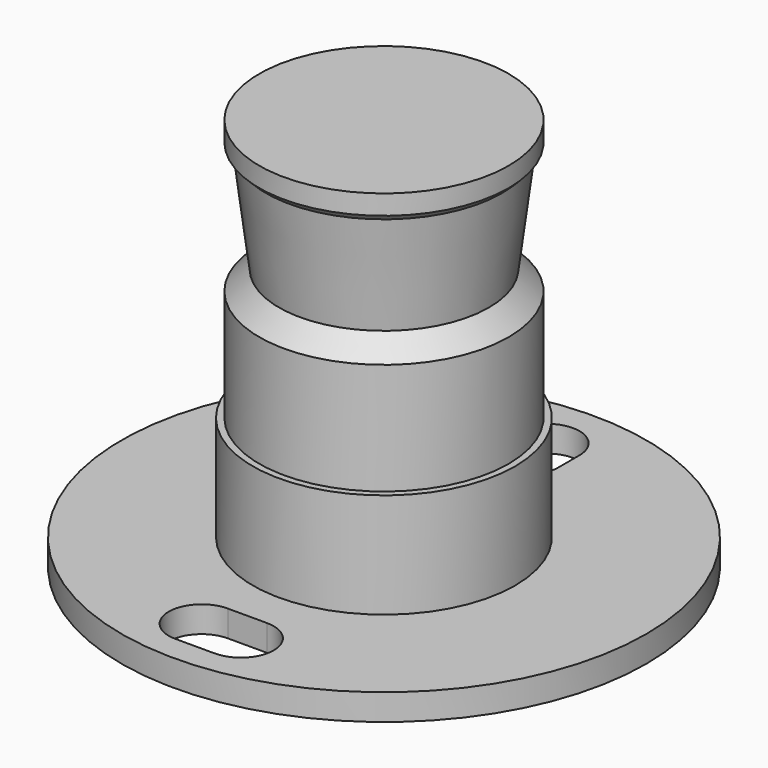
from build123d import *

# Parameters (mm, degrees)
F0_R     = 20
F1_DEPTH = 2
F4_SIZE  = 0.49999
F5_SIZE  = 1.49999


# Not quite as in the source:
# - a fillet or chamfer is up to 0.001 mm smaller than in the source, because OpenCascade refuses the exact size


with BuildPart() as f1:
    # F0 (on Top) → F1 (new body)
    with BuildSketch(Plane.XY):
        Circle(F0_R)
        with BuildLine():
            Line((-1.5, -13), (1.5, -13))
            ThreePointArc((1.5, -13), (4, -15.5), (1.5, -18))
            Line((1.5, -18), (-1.5, -18))
            ThreePointArc((-1.5, -18), (-4, -15.5), (-1.5, -13))
        make_face(mode=Mode.SUBTRACT)
        with BuildLine():
            ThreePointArc((2.5, 13.5), (0, 11), (-2.5, 13.5))
            Line((-2.5, 13.5), (-2.5, 15.5))
            ThreePointArc((-2.5, 15.5), (0, 18), (2.5, 15.5))
            Line((2.5, 15.5), (2.5, 13.5))
        make_face(mode=Mode.SUBTRACT)
    extrude(amount=F1_DEPTH)

    # F2 (on Front) → F3 (revolve)
    with BuildSketch(Plane.XZ):
        Polygon((0, 30), (0, 2), (10, 2), (10, 10), (9.5, 10), (9.5, 20), (8, 20), (9, 28), (9.5, 28), (9.5, 30), align=None)
    revolve(axis=Axis((0, 0, 44.0067852139), (0, 0, 1)))

    # F4 (size 0.5 in the source; OpenCascade refuses exactly that, so slightly less here)
    f4_edges = [f1.edges().sort_by_distance(p)[0] for p in [
        (-9.5, 0, 28),
    ]]
    chamfer(f4_edges, length=F4_SIZE)

    # F5 (size 1.5 in the source; OpenCascade refuses exactly that, so slightly less here)
    f5_edges = [f1.edges().sort_by_distance(p)[0] for p in [
        (-9.5, 0, 20),
    ]]
    chamfer(f5_edges, length=F5_SIZE)


solid = f1.part
